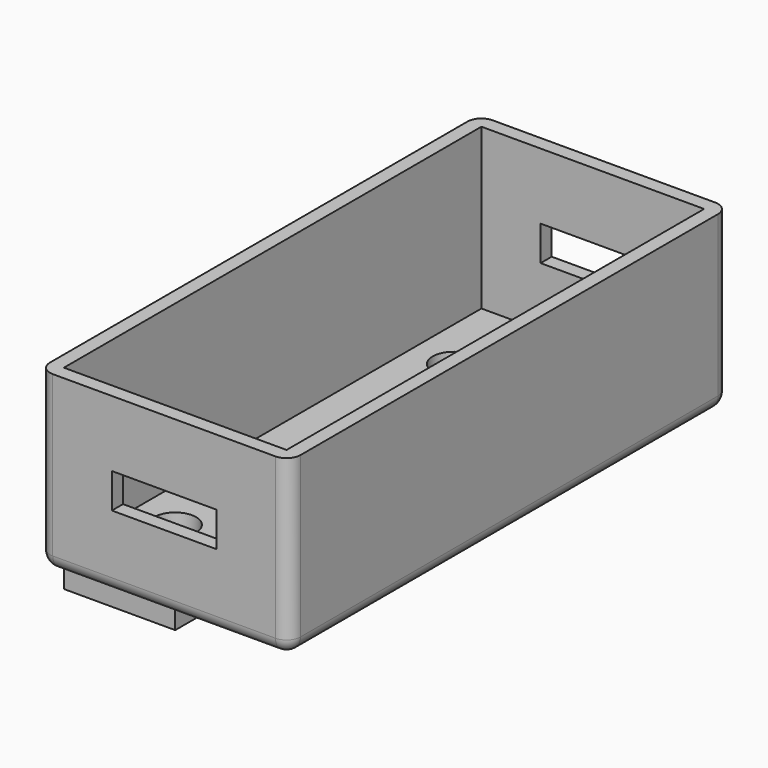
from build123d import *

# Parameters (mm, degrees)
F0_W     = 36
F0_H     = 79
F0_W_2   = 16
F0_H_2   = 75
F0_R     = 3
F1_DEPTH = 2
F2_DEPTH = 25
F0_R_2   = 1.5
F3_DEPTH = 3
F4_R     = 1.99999
F5_W     = 15
F5_H     = 5
F6_DEPTH = 100


# Not quite as in the source:
# - a fillet or chamfer is up to 0.001 mm smaller than in the source, because OpenCascade refuses the exact size


with BuildPart() as f1:
    # F0 (on Top) → F1 (new body)
    with BuildSketch(Plane.XY):
        Rectangle(F0_W, F0_H)
        Polygon((0, 37.5), (16, 37.5), (16, -37.5), (0, -37.5), (-16, -37.5), (-16, 37.5), align=None, mode=Mode.SUBTRACT)
        with Locations((8, 0)):
            Rectangle(F0_W_2, F0_H_2)
        with Locations((-8, 0)):
            Rectangle(F0_W_2, F0_H_2)
        with Locations((-10, -25)):
            Circle(F0_R, mode=Mode.SUBTRACT)
        with Locations((-10, 25)):
            Circle(F0_R, mode=Mode.SUBTRACT)
    extrude(amount=F1_DEPTH)

    # F0 (on Top) → F2 (join)
    with BuildSketch(Plane.XY):
        Rectangle(F0_W, F0_H)
        Polygon((0, 37.5), (16, 37.5), (16, -37.5), (0, -37.5), (-16, -37.5), (-16, 37.5), align=None, mode=Mode.SUBTRACT)
    extrude(amount=F2_DEPTH)

    # F0 (on Top) → F3 (join)
    with BuildSketch(Plane.XY):
        with Locations((-8, 0)):
            Rectangle(F0_W_2, F0_H_2)
        with Locations((-10, -25)):
            Circle(F0_R, mode=Mode.SUBTRACT)
        with Locations((-10, 25)):
            Circle(F0_R, mode=Mode.SUBTRACT)
        with Locations((-10, 25)):
            Circle(F0_R)
        with Locations((-10, 25)):
            Circle(F0_R_2, mode=Mode.SUBTRACT)
        with Locations((-10, -25)):
            Circle(F0_R)
        with Locations((-10, -25)):
            Circle(F0_R_2, mode=Mode.SUBTRACT)
    extrude(amount=-F3_DEPTH)

    # F4 (radius 2 in the source; OpenCascade refuses exactly that, so slightly less here)
    f4_edges = [f1.edges().sort_by_distance(p)[0] for p in [
        (-18, 0, 0),
        (0, -39.5, 0),
        (0, 39.5, 0),
        (18, 0, 0),
        (18, 39.5, 12.5),
        (-18, 39.5, 12.5),
        (-18, -39.5, 12.5),
        (18, -39.5, 12.5),
    ]]
    fillet(f4_edges, radius=F4_R)

    # F5 (on face) → F6 (cut)
    with BuildSketch(Plane.XZ.offset(39.5)):
        with Locations((0, 13.0054904148)):
            Rectangle(F5_W, F5_H)
    extrude(amount=-F6_DEPTH, mode=Mode.SUBTRACT)


solid = f1.part
